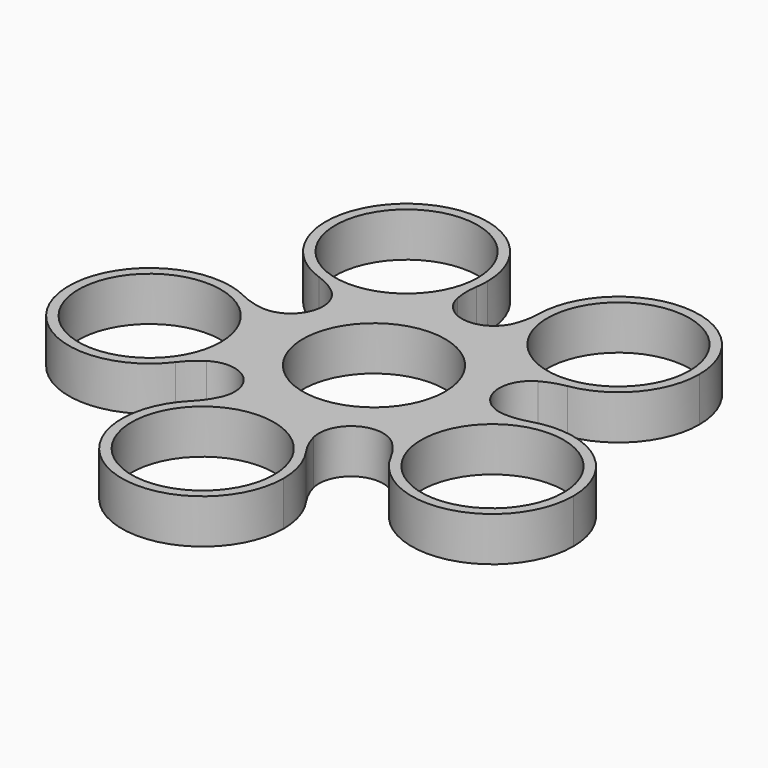
from build123d import *

# Parameters (mm, degrees)
F0_R     = 11.25
F1_DEPTH = 7
F2_R     = 5.08


# Not quite as in the source:
# - a feature names something its author has since deleted; it is built from what else it names


with BuildPart() as f1:
    # F0 (on Top) → F1 (new body)
    with BuildSketch(Plane.XY):
        with BuildLine():
            ThreePointArc((-10.2261463935, 7.6719560941), (-6.6075524932, 10.9440956877), (-2.0266855863, 12.6224215548))
            ThreePointArc((-2.0266855863, 12.6224215548), (-0.3918821811, 13.0140427744), (1.1648785444, 13.648428617))
            ThreePointArc((1.1648785444, 13.648428617), (-2.5221716271, 18.3553828089), (-3.2272094242, 24.2927794132))
            ThreePointArc((-3.2272094242, 24.2927794132), (-9.2505734905, 15.3217339628), (-19.9945367973, 14.1694216731))
            ThreePointArc((-19.9945367973, 14.1694216731), (-15.0686816006, 10.7803646784), (-12.6204597068, 5.3254617195))
            ThreePointArc((-12.6204597068, 5.3254617195), (-11.3340606288, 6.4076478244), (-10.2261463935, 7.6719560941))
        make_face()
        with BuildLine():
            ThreePointArc((12.7825888677, -0.1959648224), (12.7837153932, -0.0979852894), (12.7840909091, 0))
            ThreePointArc((12.7840909091, 0), (12.4276891989, 2.9975859532), (11.3783559826, 5.828035304))
            ThreePointArc((11.3783559826, 5.828035304), (8.3666075071, 9.666067411), (4.1364108135, 12.0964079773))
            ThreePointArc((4.1364108135, 12.0964079773), (1.0871557866, 12.7377813087), (-2.0266855863, 12.6224215548))
            ThreePointArc((-2.0266855863, 12.6224215548), (-6.6075524932, 10.9440956877), (-10.2261463935, 7.6719560941))
            ThreePointArc((-10.2261463935, 7.6719560941), (-11.7784003031, 4.9701374901), (-12.6309165595, 1.9730502372))
            ThreePointArc((-12.6309165595, 1.9730502372), (-12.4502995304, -2.9022442999), (-10.4565168586, -7.3548783509))
            ThreePointArc((-10.4565168586, -7.3548783509), (-8.3666075071, -9.666067411), (-5.7796501565, -11.4030094467))
            ThreePointArc((-5.7796501565, -11.4030094467), (-1.0871557866, -12.7377813087), (3.7636635709, -12.2175208981))
            ThreePointArc((3.7636635709, -12.2175208981), (6.6075524932, -10.9440956877), (9.0588963197, -9.0204976493))
            ThreePointArc((9.0588963197, -9.0204976493), (11.7784003031, -4.9701374901), (12.7825888677, -0.1959648224))
        make_face()
        Circle(F0_R, mode=Mode.SUBTRACT)
        with BuildLine():
            ThreePointArc((-2.0266855863, 12.6224215548), (1.0871557866, 12.7377813087), (4.1364108135, 12.0964079773))
            ThreePointArc((4.1364108135, 12.0964079773), (2.591617868, 12.7594042888), (1.1648785444, 13.648428617))
            ThreePointArc((1.1648785444, 13.648428617), (-0.3918821811, 13.0140427744), (-2.0266855863, 12.6224215548))
        make_face()
        with BuildLine():
            ThreePointArc((11.3783559826, 5.828035304), (12.4276891989, 2.9975859532), (12.7840909091, 0))
            ThreePointArc((12.7840909091, 0), (12.7837153932, -0.0979852894), (12.7825888677, -0.1959648224))
            ThreePointArc((12.7825888677, -0.1959648224), (12.935768557, 1.4780977023), (13.34039424, 3.1097310588))
            ThreePointArc((13.34039424, 3.1097310588), (12.2559919302, 4.3942624848), (11.3783559826, 5.828035304))
        make_face()
        with BuildLine():
            ThreePointArc((-12.6309165595, 1.9730502372), (-11.7784003031, 4.9701374901), (-10.2261463935, 7.6719560941))
            ThreePointArc((-10.2261463935, 7.6719560941), (-11.3340606288, 6.4076478244), (-12.6204597068, 5.3254617195))
            ThreePointArc((-12.6204597068, 5.3254617195), (-12.4981884377, 3.6488582809), (-12.6309165595, 1.9730502372))
        make_face()
        with BuildLine():
            ThreePointArc((-10.4565168586, -7.3548783509), (-12.4502995304, -2.9022442999), (-12.6309165595, 1.9730502372))
            ThreePointArc((-12.6309165595, 1.9730502372), (-12.4981884377, 3.6488582809), (-12.6204597068, 5.3254617195))
            ThreePointArc((-12.6204597068, 5.3254617195), (-18.236400325, 3.273397465), (-24.1010687164, 4.4376231269))
            ThreePointArc((-24.1010687164, 4.4376231269), (-18.9875890794, -0.2741455025), (-17.0966279638, -6.9653863197))
            ThreePointArc((-17.0966279638, -6.9653863197), (-17.7529621653, -11.0089611755), (-19.6545724794, -14.6373424139))
            ThreePointArc((-19.6545724794, -14.6373424139), (-14.9092147728, -10.999851937), (-8.9647515968, -10.3571122686))
            ThreePointArc((-8.9647515968, -10.3571122686), (-9.5964525671, -8.7992601454), (-10.4565168586, -7.3548783509))
        make_face()
        with BuildLine():
            ThreePointArc((4.1364108135, 12.0964079773), (8.3666075071, 9.666067411), (11.3783559826, 5.828035304))
            ThreePointArc((11.3783559826, 5.828035304), (12.2559919302, 4.3942624848), (13.34039424, 3.1097310588))
            ThreePointArc((13.34039424, 3.1097310588), (16.677612534, 8.0708529874), (22.1065436034, 10.5761402317))
            ThreePointArc((22.1065436034, 10.5761402317), (11.7132505099, 13.5324943754), (7.2972691493, 23.3945266088))
            ThreePointArc((7.2972691493, 23.3945266088), (5.596257378, 17.6624837194), (1.1648785444, 13.648428617))
            ThreePointArc((1.1648785444, 13.648428617), (2.591617868, 12.7594042888), (4.1364108135, 12.0964079773))
        make_face()
        with BuildLine():
            ThreePointArc((13.34039424, 3.1097310588), (12.935768557, 1.4780977023), (12.7825888677, -0.1959648224))
            ThreePointArc((12.7825888677, -0.1959648224), (11.7784003031, -4.9701374901), (9.0588963197, -9.0204976493))
            ThreePointArc((9.0588963197, -9.0204976493), (7.9665017598, -10.2982392034), (7.0799385192, -11.7265091268))
            ThreePointArc((7.0799385192, -11.7265091268), (12.8295030243, -13.3673213445), (16.8898047449, -17.7563652803))
            ThreePointArc((16.8898047449, -17.7563652803), (16.4897604244, -6.9581924862), (24.5044971566, 0.2891909218))
            ThreePointArc((24.5044971566, 0.2891909218), (18.52735887, 0.1356505859), (13.34039424, 3.1097310588))
        make_face()
        with BuildLine():
            ThreePointArc((7.0799385192, -11.7265091268), (7.9665017598, -10.2982392034), (9.0588963197, -9.0204976493))
            ThreePointArc((9.0588963197, -9.0204976493), (6.6075524932, -10.9440956877), (3.7636635709, -12.2175208981))
            ThreePointArc((3.7636635709, -12.2175208981), (5.4031267709, -11.8458896701), (7.0799385192, -11.7265091268))
        make_face()
        with BuildLine():
            ThreePointArc((-8.9647515968, -10.3571122686), (-7.3324230712, -10.7589243367), (-5.7796501565, -11.4030094467))
            ThreePointArc((-5.7796501565, -11.4030094467), (-8.3666075071, -9.666067411), (-10.4565168586, -7.3548783509))
            ThreePointArc((-10.4565168586, -7.3548783509), (-9.5964525671, -8.7992601454), (-8.9647515968, -10.3571122686))
        make_face()
        with BuildLine():
            ThreePointArc((7.0799385192, -11.7265091268), (5.4031267709, -11.8458896701), (3.7636635709, -12.2175208981))
            ThreePointArc((3.7636635709, -12.2175208981), (-1.0871557866, -12.7377813087), (-5.7796501565, -11.4030094467))
            ThreePointArc((-5.7796501565, -11.4030094467), (-7.3324230712, -10.7589243367), (-8.9647515968, -10.3571122686))
            ThreePointArc((-8.9647515968, -10.3571122686), (-8.7485436062, -16.3323119169), (-11.6680702077, -21.5501774915))
            ThreePointArc((-11.6680702077, -21.5501774915), (-1.5220181013, -17.8328938321), (7.8473429707, -23.2157967899))
            ThreePointArc((7.8473429707, -23.2157967899), (5.8542801254, -17.5786470467), (7.0799385192, -11.7265091268))
        make_face()
        with BuildLine():
            ThreePointArc((41.0522516366, -11.9283299763), (35.8615118695, -1.64368128), (24.5044971566, 0.2891909218))
            ThreePointArc((24.5044971566, 0.2891909218), (16.4897604244, -6.9581924862), (16.8898047449, -17.7563652803))
            ThreePointArc((16.8898047449, -17.7563652803), (31.2657466808, -24.3560191752), (41.0522516366, -11.9283299763))
        make_face()
        with Locations((28.2681607275, -11.9283299763)):
            Circle(F0_R, mode=Mode.SUBTRACT)
        with BuildLine():
            ThreePointArc((10.1749170211, -30.5706751408), (9.5791410589, -26.713479381), (7.8473429707, -23.2157967899))
            ThreePointArc((7.8473429707, -23.2157967899), (-1.5220181013, -17.8328938321), (-11.6680702077, -21.5501774915))
            ThreePointArc((-11.6680702077, -21.5501774915), (-7.4888883409, -42.3868237193), (10.1749170211, -30.5706751408))
        make_face()
        with Locations((-2.6091738879, -30.5706751408)):
            Circle(F0_R, mode=Mode.SUBTRACT)
        with BuildLine():
            ThreePointArc((-17.0966279638, -6.9653863197), (-18.9875890794, -0.2741455025), (-24.1010687164, 4.4376231269))
            ThreePointArc((-24.1010687164, 4.4376231269), (-42.3310184032, -9.8676306196), (-19.6545724794, -14.6373424139))
            ThreePointArc((-19.6545724794, -14.6373424139), (-17.7529621653, -11.0089611755), (-17.0966279638, -6.9653863197))
        make_face()
        with Locations((-29.8807188729, -6.9653863197)):
            Circle(F0_R, mode=Mode.SUBTRACT)
        with BuildLine():
            ThreePointArc((-19.9945367973, 14.1694216731), (-9.2505734905, 15.3217339628), (-3.2272094242, 24.2927794132))
            ThreePointArc((-3.2272094242, 24.2927794132), (-3.112386187, 25.2763361411), (-3.0740350747, 26.2658296504))
            ThreePointArc((-3.0740350747, 26.2658296504), (-23.2929335971, 36.6656669628), (-19.9945367973, 14.1694216731))
        make_face()
        with Locations((-15.8581259838, 26.2658296504)):
            Circle(F0_R, mode=Mode.SUBTRACT)
        with BuildLine():
            ThreePointArc((7.2972691493, 23.3945266088), (11.7132505099, 13.5324943754), (22.1065436034, 10.5761402317))
            ThreePointArc((22.1065436034, 10.5761402317), (29.8097684265, 14.9062868395), (32.8639489261, 23.1985617864))
            ThreePointArc((32.8639489261, 23.1985617864), (20.1778433064, 35.9822771796), (7.2972691493, 23.3945266088))
        make_face()
        with Locations((20.079858017, 23.1985617864)):
            Circle(F0_R, mode=Mode.SUBTRACT)
    extrude(amount=F1_DEPTH)

    # F2
    f2_edges = [f1.edges().sort_by_distance(p)[0] for p in [
        (7.079939, -11.726509, 3.5),
        (-8.964752, -10.357112, 3.5),
        (-12.62046, 5.325462, 3.5),
        (1.164879, 13.648429, 3.5),
        (13.340394, 3.109731, 3.5),
    ]]
    fillet(f2_edges, radius=F2_R)


solid = f1.part
